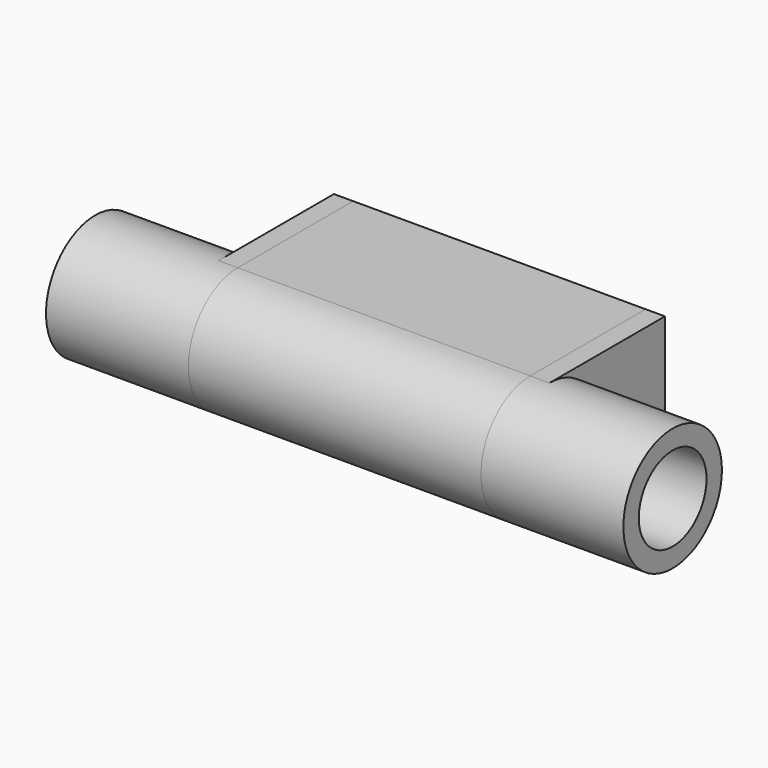
from build123d import *

# Parameters (mm, degrees)
F0_W          = 37.592
F0_H          = 5.08
F2_W          = 77.216
F2_H          = 5.08
F3_ANGLE_BACK = 90
F3_ANGLE      = 180
F4_W          = 77.216
F4_H          = 5.08
F5_DEPTH      = 38.1
F7_DEPTH      = 5.08
F9_DEPTH      = 5.08


with BuildPart() as f1:
    # F0 (on Top) → F1 (revolve)
    with BuildSketch(Plane.XY):
        with Locations((-57.404, 13.716)):
            Rectangle(F0_W, F0_H)
    revolve(axis=Axis((-4.8519736156, 0, 0), (1, 0, 0)))

    # F6 (on face) → F7 (join)
    with BuildSketch(Plane.YZ.offset(-38.608)):
        with BuildLine():
            Line((38.1, 16.256), (0, 16.256))
            ThreePointArc((0, 16.256), (11.494727835, 11.494727835), (16.256, 0))
            ThreePointArc((16.256, 0), (11.494727835, -11.494727835), (0, -16.256))
            Line((0, -16.256), (38.1, -16.256))
            Line((38.1, -16.256), (38.1, 16.256))
        make_face()
    extrude(amount=-F7_DEPTH)


with BuildPart() as f1b:
    # F0 (on Top) → F1, piece 2 (revolve)
    with BuildSketch(Plane.XY):
        with Locations((57.404, 13.716)):
            Rectangle(F0_W, F0_H)
    revolve(axis=Axis((-4.8519736156, 0, 0), (1, 0, 0)))

    # F8 (on face) → F9 (join)
    with BuildSketch(Plane(origin=(38.608, 0, 0), x_dir=(0, -1, 0), z_dir=(-1, 0, 0))):
        with BuildLine():
            ThreePointArc((0, -16.256), (-16.256, 0), (0, 16.256))
            Line((0, 16.256), (-38.1, 16.256))
            Line((-38.1, 16.256), (-38.1, -16.256))
            Line((-38.1, -16.256), (0, -16.256))
        make_face()
    extrude(amount=-F9_DEPTH)


with BuildPart() as f3:
    # F2 (on Top) → F3 (revolve)
    with BuildSketch(Plane.XY, mode=Mode.PRIVATE) as f3_sk:
        with Locations((0, -13.716)):
            Rectangle(F2_W, F2_H)
    revolve(f3_sk.sketch.rotate(Axis((-9.3715274706, 0, 0), (1, 0, 0)), -F3_ANGLE_BACK), axis=Axis((-9.3715274706, 0, 0), (1, 0, 0)), revolution_arc=F3_ANGLE)


with BuildPart() as f5:
    # F4 (on Front) → F5 (new body)
    with BuildSketch(Plane.XZ):
        with Locations((0, 13.716)):
            Rectangle(F4_W, F4_H)
    extrude(amount=-F5_DEPTH)


with BuildPart() as f5b:
    # F4 (on Front) → F5, piece 2 (new body)
    with BuildSketch(Plane.XZ):
        with Locations((0, -13.716)):
            Rectangle(F4_W, F4_H)
    extrude(amount=-F5_DEPTH)


solid = Compound([f1.part, f1b.part, f3.part, f5.part, f5b.part])
